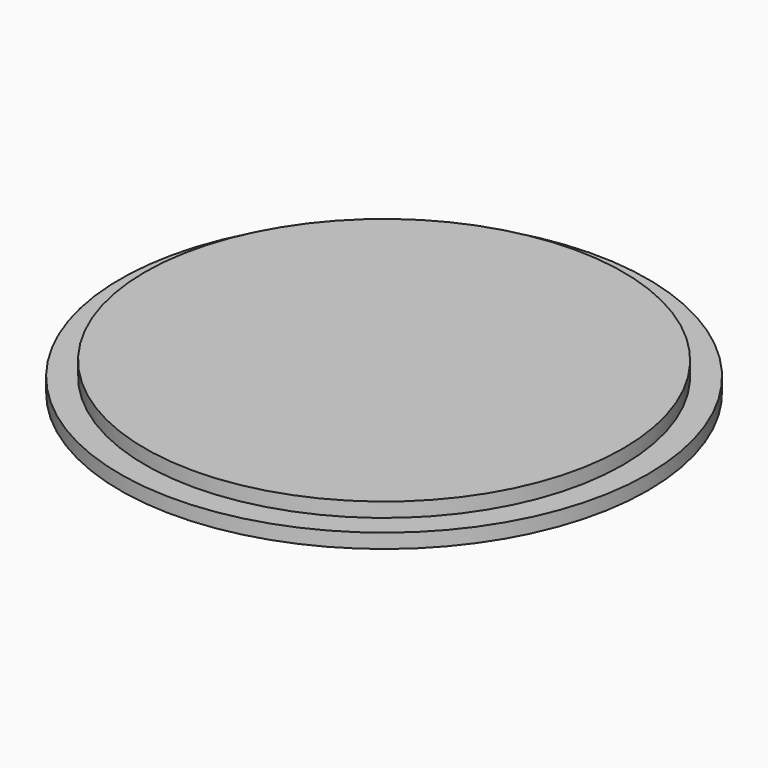
from build123d import *

# Parameters (mm, degrees)
F0_R     = 12.65
F1_DEPTH = 1.524
F2_R     = 13.97
F3_DEPTH = 0.762
F4_W     = 5.08
F4_H     = 1.524
F6_W     = 5.08000508
F6_H     = 1.5265774739
F7_DEPTH = 0.254
F8_R     = 0.25399


# Not quite as in the source:
# - a fillet or chamfer is up to 0.001 mm smaller than in the source, because OpenCascade refuses the exact size


with BuildPart() as f1:
    # F0 (on Top) → F1 (new body)
    with BuildSketch(Plane.XY):
        Circle(F0_R)
    extrude(amount=F1_DEPTH)

    # F2 (on Top) → F3 (join)
    with BuildSketch(Plane.XY):
        Circle(F2_R)
    extrude(amount=F3_DEPTH)

    # F4 (on Front) → F5 (revolve, cut)
    with BuildSketch(Plane.XZ):
        Rectangle(F4_W, F4_H)
    revolve(axis=Axis((0, 0, -0.762), (-1, 0, 0)), mode=Mode.SUBTRACT)

    # F6 (on Top) → F7 (join)
    with BuildSketch(Plane.XY):
        Rectangle(F6_W, F6_H)
    extrude(amount=F7_DEPTH)

    # F8 (radius 0.254 in the source; OpenCascade refuses exactly that, so slightly less here)
    f8_edges = [f1.edges().sort_by_distance(p)[0] for p in [
        (0, 0.763289, 0.254),
        (0, -0.763289, 0.254),
    ]]
    fillet(f8_edges, radius=F8_R)


solid = f1.part
